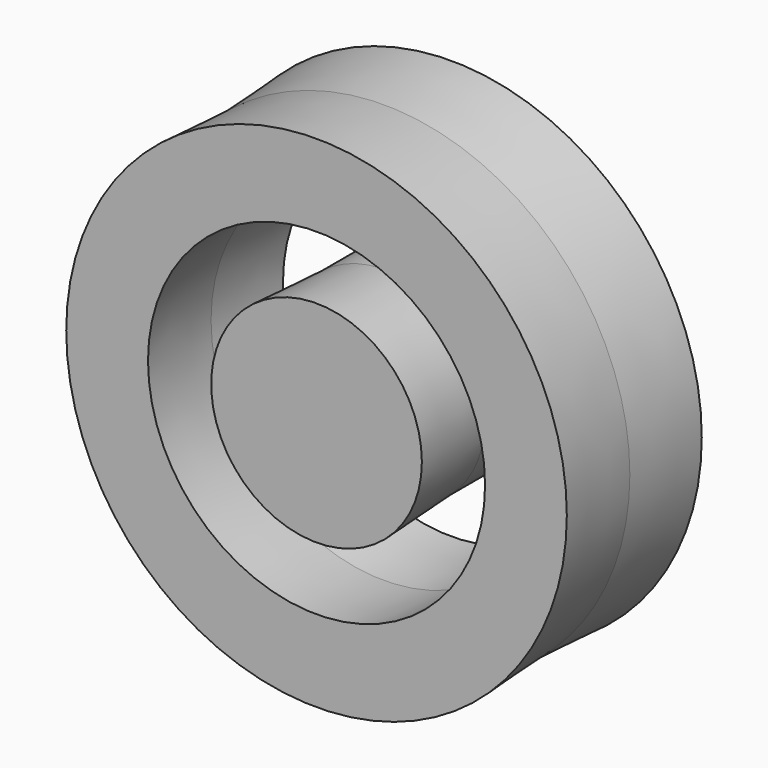
from build123d import *

# Parameters (mm, degrees)
F0_R          = 74.0552381164
F0_R_2        = 52.091292541
F1_DEPTH      = 25.4
F1_TAPER      = -3
F1_DEPTH_BACK = 25.4
F1_TAPER_BACK = -3
F4_R          = 30.393781641
F5_DEPTH      = 25.4
F5_TAPER      = -3
F5_DEPTH_BACK = 25.4


# Not quite as in the source:
# - the program builds the solid bodies; features that only make, move or delete a surface that nothing else refers to are left out


with BuildPart() as f1:
    # F0 (on Front) → F1 (new body, two sides)
    with BuildSketch(Plane.XZ) as f1_sk:
        Circle(F0_R)
        Circle(F0_R_2, mode=Mode.SUBTRACT)
    extrude(amount=F1_DEPTH, taper=F1_TAPER)
    extrude(f1_sk.sketch, amount=-F1_DEPTH_BACK, taper=F1_TAPER_BACK)


with BuildPart() as f5:
    # F4 (on Front) → F5 (new body, two sides)
    with BuildSketch(Plane.XZ) as f5_sk:
        Circle(F4_R)
    extrude(amount=F5_DEPTH, taper=F5_TAPER)
    extrude(f5_sk.sketch, amount=-F5_DEPTH_BACK)


solid = Compound([f1.part, f5.part])
